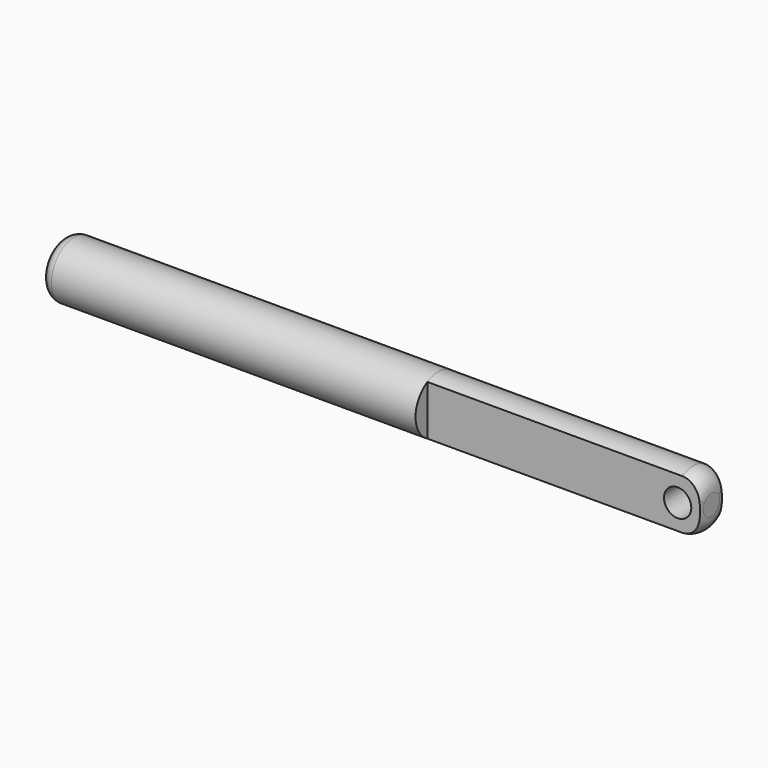
from build123d import *

# Parameters (mm, degrees)
F0_R        = 12.5
F1_DEPTH    = 165
F2_R        = 5
F5_DEPTH    = 120
F6_R        = 6
F7_DEPTH    = 18.501
F8_T2_ANGLE = 240.7472216417
F8_T4_ANGLE = 240.7472216417


# Not quite as in the source:
# - a fillet or chamfer that OpenCascade refuses, or shapes differently, is made with other operations: its cross-section is extruded or revolved along the edge and cut away or added


with BuildPart() as f1:
    # F0 (on Right) → F1 (new body)
    with BuildSketch(Plane.YZ):
        with Locations((0, 79.4712570496)):
            Circle(F0_R)
    extrude(amount=-F1_DEPTH)

    # F2
    f2_edges = [f1.edges().sort_by_distance(p)[0] for p in [
        (-165, -12.5, 79.471257),
    ]]
    fillet(f2_edges, radius=F2_R)

    # F4 (on face) → F5 (join)
    with BuildSketch(Plane.YZ):
        with BuildLine():
            ThreePointArc((6, 90.4371131493), (0, 91.9712570496), (-6, 90.4371131493))
            Line((-6, 90.4371131493), (-6, 68.5054009499))
            ThreePointArc((-6, 68.5054009499), (0, 66.9712570496), (6, 68.5054009499))
            Line((6, 68.5054009499), (6, 90.4371131493))
        make_face()
    extrude(amount=F5_DEPTH)

    # F6 (on face) → F7 (cut, through all)
    with BuildSketch(Plane.XZ.offset(6)):
        with Locations((110, 79.4712570496)):
            Circle(F6_R)
    extrude(amount=-F7_DEPTH, mode=Mode.SUBTRACT)

    # F8: fillet of radius 8 on 2 edges, made by hand

    # F8_s1 → F8_t2 (revolve, cut)
    with BuildSketch(Plane(origin=(0, 34.6682356906, 59.1529818038), x_dir=(1, 0, 0), z_dir=(0, 0.5056364556, 0.8627466458))):
        with BuildLine():
            ThreePointArc((112, -52.6835647356), (117.6568542495, -50.3404189851), (120, -44.6835647356))
            Line((120, -44.6835647356), (120, -52.6835647356))
            Line((120, -52.6835647356), (112, -52.6835647356))
        make_face()
    revolve(axis=Axis((120, 0, 79.4712570496), (1, 0, 0)), revolution_arc=F8_T2_ANGLE, mode=Mode.SUBTRACT)

    # F8_s3 → F8_t4 (revolve, cut)
    with BuildSketch(Plane(origin=(0, 34.6682356906, 59.1529818038), x_dir=(1, 0, 0), z_dir=(0, -0.5056364556, -0.8627466458))):
        with BuildLine():
            ThreePointArc((112, 27.6835647356), (117.6568542495, 30.0267104861), (120, 35.6835647356))
            Line((120, 35.6835647356), (120, 27.6835647356))
            Line((120, 27.6835647356), (112, 27.6835647356))
        make_face()
    revolve(axis=Axis((120, 0, 79.4712570496), (1, 0, 0)), revolution_arc=F8_T4_ANGLE, mode=Mode.SUBTRACT)


solid = f1.part
